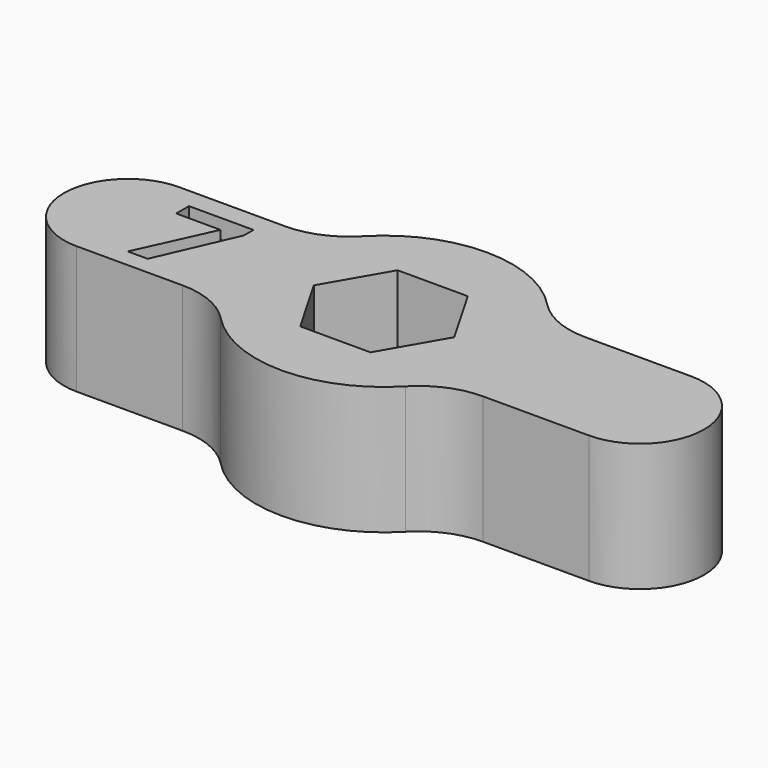
from build123d import *

# Parameters (mm, degrees)
F1_DEPTH     = 8
F2_TEXT_SIZE = 7.8653974924
F3_DEPTH     = 1.2
F4_R         = 5
F5_SIZE      = 0.5


# Not quite as in the source:
# - Text() gives the source's letters only with a copy of the font that has no kerning and outlines rounded to 1/6400 em; it was checked with that copy


with BuildPart() as f1:
    # F0 (on Top) → F1 (new body)
    with BuildSketch(Plane.XY):
        with BuildLine():
            ThreePointArc((-11.3450387246, 0.1292171509), (-12.4168354943, 4.1292171509), (-11.3450387246, 8.1292171509))
            Line((-11.3450387246, 8.1292171509), (-20.4168354943, 8.1292171509))
            ThreePointArc((-20.4168354943, 8.1292171509), (-24.4168354943, 4.1292171509), (-20.4168354943, 0.1292171509))
            Line((-20.4168354943, 0.1292171509), (-11.3450387246, 0.1292171509))
        make_face()
        with BuildLine():
            ThreePointArc((2.5113677359, 0.1292171509), (3.310571116, 2.0586647901), (3.5831645057, 4.1292171509))
            ThreePointArc((3.5831645057, 4.1292171509), (3.310571116, 6.1997695118), (2.5113677359, 8.1292171509))
            ThreePointArc((2.5113677359, 8.1292171509), (-4.4168354943, 12.1292171509), (-11.3450387246, 8.1292171509))
            ThreePointArc((-11.3450387246, 8.1292171509), (-12.4168354943, 4.1292171509), (-11.3450387246, 0.1292171509))
            ThreePointArc((-11.3450387246, 0.1292171509), (-4.4168354943, -3.8707828491), (2.5113677359, 0.1292171509))
        make_face()
        Polygon((-2.2229044714, 7.9292171509), (-0.0289734485, 4.1292171509), (-2.2229044714, 0.3292171509), (-6.6107665173, 0.3292171509), (-8.8046975402, 4.1292171509), (-6.6107665173, 7.9292171509), align=None, mode=Mode.SUBTRACT)
        with BuildLine():
            ThreePointArc((2.5113677359, 8.1292171509), (3.310571116, 6.1997695118), (3.5831645057, 4.1292171509))
            ThreePointArc((3.5831645057, 4.1292171509), (3.310571116, 2.0586647901), (2.5113677359, 0.1292171509))
            Line((2.5113677359, 0.1292171509), (11.5831645057, 0.1292171509))
            ThreePointArc((11.5831645057, 0.1292171509), (15.5831645057, 4.1292171509), (11.5831645057, 8.1292171509))
            Line((11.5831645057, 8.1292171509), (2.5113677359, 8.1292171509))
        make_face()
    extrude(amount=F1_DEPTH)

    # F2 (on face) → F3 (cut)
    with BuildSketch(Plane.XY.offset(8)):
        with Locations((-19.00204923, 1.2564882636)):
            Text('7', F2_TEXT_SIZE, font='Open Sans', font_style=FontStyle.BOLD, text_align=(TextAlign.LEFT, TextAlign.BOTTOM))
    extrude(amount=-F3_DEPTH, mode=Mode.SUBTRACT)

    # F4
    f4_edges = [f1.edges().sort_by_distance(p)[0] for p in [
        (2.511368, 0.129217, 4),
        (-11.345039, 0.129217, 4),
        (2.511368, 8.129217, 4),
        (-11.345039, 8.129217, 4),
    ]]
    fillet(f4_edges, radius=F4_R)

    # F5
    f5_edges = [f1.edges().sort_by_distance(p)[0] for p in [
        (-4.416835, 0.329217, 0),
        (-7.707732, 2.229217, 0),
        (-7.707732, 6.029217, 0),
        (-4.416835, 7.929217, 0),
        (-1.125939, 6.029217, 0),
        (-1.125939, 2.229217, 0),
    ]]
    chamfer(f5_edges, length=F5_SIZE)


solid = f1.part
